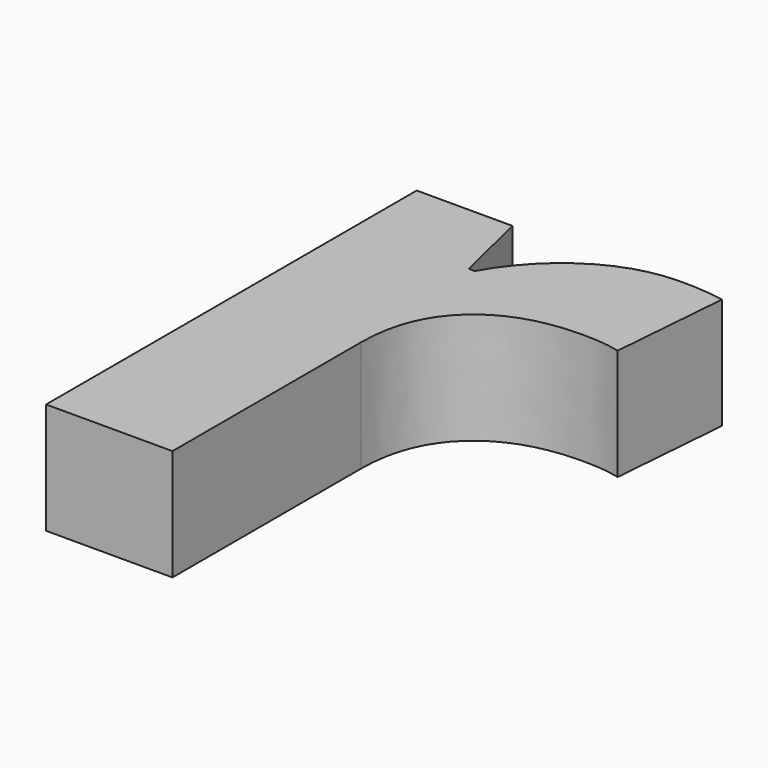
from build123d import *

# Parameters (mm, degrees)
F0_TEXT_SIZE = 76.2947990249
F1_DEPTH     = 10


# Not quite as in the source:
# - Text() gives the source's letters only with a copy of the font that has no kerning and outlines rounded to 1/6400 em; it was checked with that copy


with BuildPart() as f1:
    # F0 (on Top) → F1 (new body)
    with BuildSketch(Plane.XY):
        with Locations((0, 0)):
            Text('r', F0_TEXT_SIZE, font='Open Sans', font_style=FontStyle.BOLD, text_align=(TextAlign.LEFT, TextAlign.BOTTOM))
    extrude(amount=F1_DEPTH)


solid = f1.part
